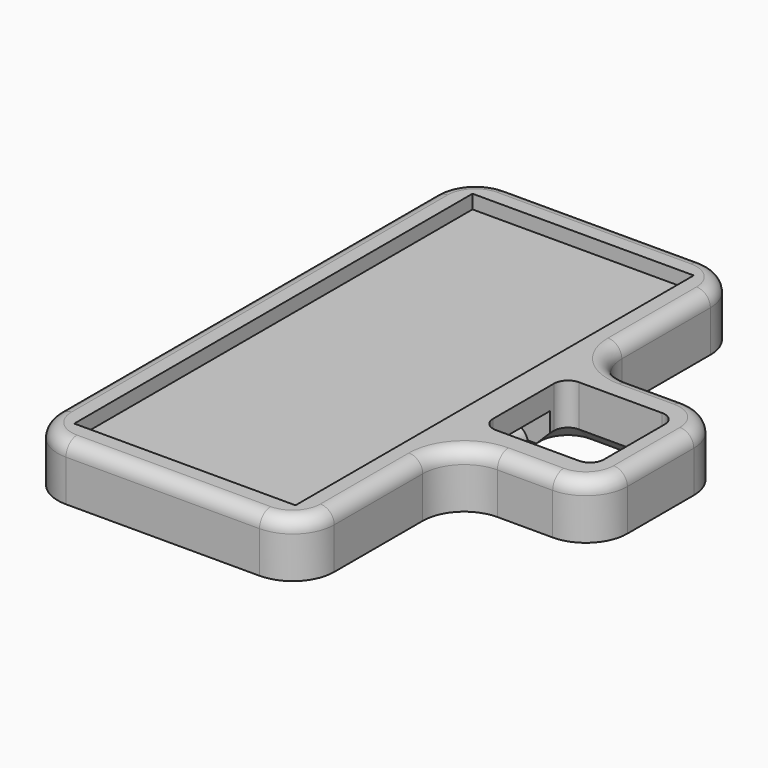
from build123d import *

# Parameters (mm, degrees)
F0_W         = 16
F0_H         = 36
F1_DEPTH     = 4
F2_DEPTH     = 3
F3_W         = 4.8
F3_H         = 1.6
F4_DEPTH     = 20.1
F5_T1_DEPTH  = 5.5
F5_T3_DEPTH  = 6
F5_T6_ANGLE  = 90
F5_T8_ANGLE  = 90
F5_T10_ANGLE = 90
F5_T12_ANGLE = 90
F6_T1_DEPTH  = 4.8
F7_R         = 1


# Not quite as in the source:
# - a fillet or chamfer that OpenCascade refuses, or shapes differently, is made with other operations: its cross-section is extruded or revolved along the edge and cut away or added


with BuildPart() as f1:
    # F0 (on Top) → F1 (new body)
    with BuildSketch(Plane.XY):
        with BuildLine():
            ThreePointArc((10, 17), (9.1213203436, 19.1213203436), (7, 20))
            Line((7, 20), (-7, 20))
            ThreePointArc((-7, 20), (-9.1213203436, 19.1213203436), (-10, 17))
            Line((-10, 17), (-10, -17))
            ThreePointArc((-10, -17), (-9.1213203436, -19.1213203436), (-7, -20))
            Line((-7, -20), (7, -20))
            ThreePointArc((7, -20), (9.1213203436, -19.1213203436), (10, -17))
            Line((10, -17), (10, -9))
            ThreePointArc((10, -9), (10.8786796564, -6.8786796564), (13, -6))
            Line((13, -6), (17, -6))
            ThreePointArc((17, -6), (19.1213203436, -5.1213203436), (20, -3))
            Line((20, -3), (20, 3))
            ThreePointArc((20, 3), (19.1213203436, 5.1213203436), (17, 6))
            Line((17, 6), (13, 6))
            ThreePointArc((13, 6), (10.8786796564, 6.8786796564), (10, 9))
            Line((10, 9), (10, 17))
        make_face()
        Rectangle(F0_W, F0_H, mode=Mode.SUBTRACT)
        with BuildLine():
            ThreePointArc((10.1, 2.75), (10.3928932188, 3.4571067812), (11.1, 3.75))
            Line((11.1, 3.75), (17.1, 3.75))
            ThreePointArc((17.1, 3.75), (17.8071067812, 3.4571067812), (18.1, 2.75))
            Line((18.1, 2.75), (18.1, -2.75))
            ThreePointArc((18.1, -2.75), (17.8071067812, -3.4571067812), (17.1, -3.75))
            Line((17.1, -3.75), (11.1, -3.75))
            ThreePointArc((11.1, -3.75), (10.3928932188, -3.4571067812), (10.1, -2.75))
            Line((10.1, -2.75), (10.1, 2.75))
        make_face(mode=Mode.SUBTRACT)
    extrude(amount=F1_DEPTH)

    # F0 (on Top) → F2 (join)
    with BuildSketch(Plane.XY):
        Rectangle(F0_W, F0_H)
    extrude(amount=F2_DEPTH)

    # F3 (on face) → F4 (cut, through all)
    with BuildSketch(Plane(origin=(-10, 0, 0), x_dir=(0, -1, 0), z_dir=(-1, 0, 0))):
        with Locations((0, 1.6)):
            Rectangle(F3_W, F3_H)
    extrude(amount=-F4_DEPTH, mode=Mode.SUBTRACT)

    # F5: chamfer of 1 on 1 edges, made by hand

    # F5_s2 → F5_t1 (cut)
    with BuildSketch(Plane.XZ.offset(-2.75)):
        Polygon((19.1, 0), (18.1, 1), (18.1, 0), align=None)
        Polygon((9.1, 0), (10.1, 1), (10.1, 0), align=None)
    extrude(amount=F5_T1_DEPTH, mode=Mode.SUBTRACT)

    # F5_s4 → F5_t3 (cut)
    with BuildSketch(Plane.YZ.offset(11.1)):
        Polygon((-4.75, 0), (-3.75, 1), (-3.75, 0), align=None)
        Polygon((4.75, 0), (3.75, 1), (3.75, 0), align=None)
    extrude(amount=F5_T3_DEPTH, mode=Mode.SUBTRACT)

    # F5_s5 → F5_t6 (revolve, cut)
    with BuildSketch(Plane.YZ.offset(17.1)):
        Polygon((4.75, 0), (3.75, 1), (3.75, 0), align=None)
    revolve(axis=Axis((17.1, 2.75, 0), (0, 0, -1)), revolution_arc=F5_T6_ANGLE, mode=Mode.SUBTRACT)

    # F5_s7 → F5_t8 (revolve, cut)
    with BuildSketch(Plane.XZ.offset(2.75)):
        Polygon((19.1, 0), (18.1, 1), (18.1, 0), align=None)
    revolve(axis=Axis((17.1, -2.75, 0), (0, 0, -1)), revolution_arc=F5_T8_ANGLE, mode=Mode.SUBTRACT)

    # F5_s9 → F5_t10 (revolve, cut)
    with BuildSketch(Plane.YZ.offset(11.1)):
        Polygon((-4.75, 0), (-3.75, 1), (-3.75, 0), align=None)
    revolve(axis=Axis((11.1, -2.75, 0), (0, 0, -1)), revolution_arc=F5_T10_ANGLE, mode=Mode.SUBTRACT)

    # F5_s11 → F5_t12 (revolve, cut)
    with BuildSketch(Plane.XZ.offset(-2.75)):
        Polygon((9.1, 0), (10.1, 1), (10.1, 0), align=None)
    revolve(axis=Axis((11.1, 2.75, 0), (0, 0, -1)), revolution_arc=F5_T12_ANGLE, mode=Mode.SUBTRACT)

    # F6: fillet of radius 1 on 1 edges, made by hand

    # F6_s2 → F6_t1 (cut)
    with BuildSketch(Plane.XZ.offset(-2.4)):
        with BuildLine():
            ThreePointArc((8.1928932188, -0.9071067812), (8.4096659701, 0.1826834324), (7.4857864376, 0.8))
            Line((7.4857864376, 0.8), (9.9, 0.8))
            Line((9.9, 0.8), (8.1928932188, -0.9071067812))
        make_face()
    extrude(amount=F6_T1_DEPTH, mode=Mode.SUBTRACT)

    # F7
    f7_edges = [f1.edges().sort_by_distance(p)[0] for p in [
        (-10, 0, 4),
    ]]
    fillet(f7_edges, radius=F7_R)


solid = f1.part
